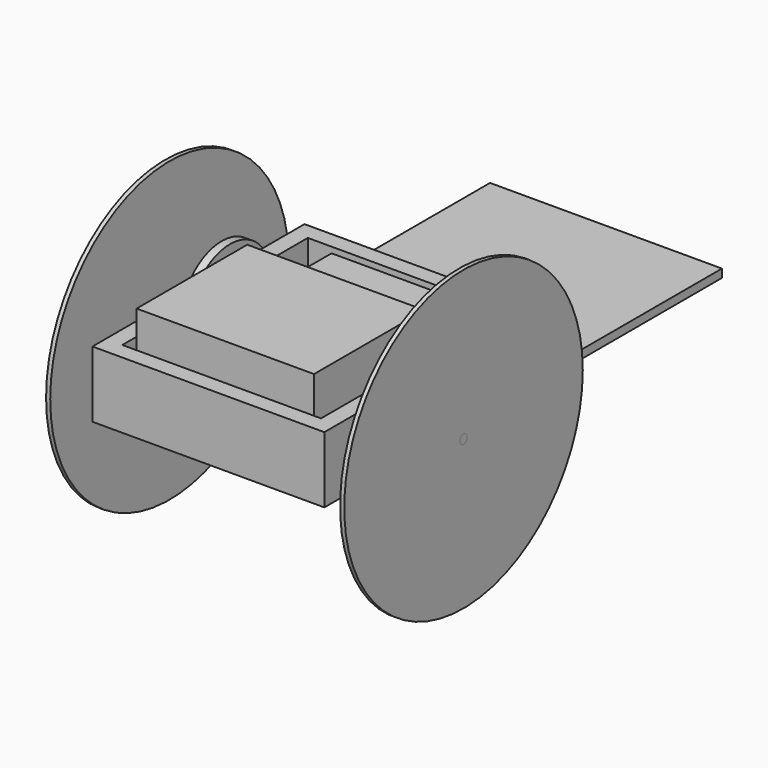
from build123d import *

# Parameters (mm, degrees)
F0_W           = 88.9
F0_H           = 101.6
F0_W_2         = 76.2
F0_H_2         = 88.9
F1_DEPTH       = 25.4
F2_DEPTH       = 3.175
F3_W           = 88.9
F3_H           = 3.175
F4_DEPTH       = 76.2
F5_W           = 47.999904
F5_H           = 25.0000008
F6_DEPTH       = 15.0114
F5_W_2         = 68.000118
F5_H_2         = 52.999894
F7_DEPTH       = 26.0096
F8_R           = 1.7859375
F9_DEPTH       = 6.35
F10_R          = 1.7859375
F11_DEPTH      = 6.35
F12_DEPTH      = 57.15
F12_DEPTH_BACK = 57.15
F15_R          = 57.15
F15_R_2        = 1.7859375
F16_DEPTH      = 1.5875
F17_R          = 57.15
F17_R_2        = 1.7859375
F18_DEPTH      = 1.5875
F20_R          = 1.7859375
F21_DEPTH      = 3.175
F22_R          = 5.0000027
F22_R_2        = 1.7859375
F23_DEPTH      = 3.175
F20_R_2        = 19.99996
F24_DEPTH      = 3.175
F25_DEPTH      = 3.175
F26_DEPTH      = 3.175


# Not quite as in the source:
# - a length typed as a fraction of an inch, garbled in the dataset ("3 / 203.2 mm" for 3/8 in), is restored


with BuildPart() as f1:
    # F0 (on Top) → F1 (new body)
    with BuildSketch(Plane.XY):
        Rectangle(F0_W, F0_H)
        Rectangle(F0_W_2, F0_H_2, mode=Mode.SUBTRACT)
    extrude(amount=F1_DEPTH)

    # F0 (on Top) → F2 (join)
    with BuildSketch(Plane.XY):
        Rectangle(F0_W_2, F0_H_2)
    extrude(amount=F2_DEPTH)

    # F8 (on face) → F9 (cut)
    with BuildSketch(Plane(origin=(-44.45, 0, 0), x_dir=(0, -1, 0), z_dir=(-1, 0, 0))):
        with Locations((0, 6.5484375)):
            Circle(F8_R)
    extrude(amount=-F9_DEPTH, mode=Mode.SUBTRACT)

    # F10 (on face) → F11 (cut)
    with BuildSketch(Plane.YZ.offset(44.45)):
        with Locations((0, 6.5484375)):
            Circle(F10_R)
    extrude(amount=-F11_DEPTH, mode=Mode.SUBTRACT)

    # F0 (on Top) → F26 (join)
    with BuildSketch(Plane.XY):
        with Locations((0, 95.25)):
            Rectangle(F0_W, F0_H_2)
    extrude(amount=F26_DEPTH)


with BuildPart() as f4:
    # F3 (on face) → F4 (new body)
    with BuildSketch(Plane.YZ.offset(-38.1)):
        with Locations((0, 10.715625)):
            Rectangle(F3_W, F3_H)
    extrude(amount=F4_DEPTH)


with BuildPart() as f6:
    # F5 (on face) → F6 (new body)
    with BuildSketch(Plane.XY.offset(12.303125)):
        with Locations((0, 25.7093309629)):
            Rectangle(F5_W, F5_H)
    extrude(amount=F6_DEPTH)


with BuildPart() as f7:
    # F5 (on face) → F7 (new body)
    with BuildSketch(Plane.XY.offset(12.303125)):
        with Locations((0, -16.2006690371)):
            Rectangle(F5_W_2, F5_H_2)
    extrude(amount=F7_DEPTH)


with BuildPart() as f12:
    # F8 (on face) → F12 (new body, two sides)
    with BuildSketch(Plane(origin=(-44.45, 0, 0), x_dir=(0, -1, 0), z_dir=(-1, 0, 0))) as f12_sk:
        with Locations((0, 6.5484375)):
            Circle(F8_R)
    extrude(amount=-F12_DEPTH)
    extrude(f12_sk.sketch, amount=F12_DEPTH_BACK)


with BuildPart() as f12_1:
    # F13: moved
    add(f12.part.moved(Location((38.1, 0, 0))))


with BuildPart() as f12_2:
    # F14: moved
    add(f12_1.part.moved(Location((6.35, 0, 0))))


with BuildPart() as f16:
    # F15 (on face) → F16 (new body)
    with BuildSketch(Plane.YZ.offset(57.15)):
        with Locations((0, 6.5484375)):
            Circle(F15_R)
        with Locations((0, 6.5484375)):
            Circle(F15_R_2, mode=Mode.SUBTRACT)
    extrude(amount=-F16_DEPTH)


with BuildPart() as f18:
    # F17 (on face) → F18 (new body)
    with BuildSketch(Plane(origin=(-57.15, 0, 0), x_dir=(0, -1, 0), z_dir=(-1, 0, 0))):
        with Locations((0, 6.5484375)):
            Circle(F17_R)
        with Locations((0, 6.5484375)):
            Circle(F17_R_2, mode=Mode.SUBTRACT)
    extrude(amount=-F18_DEPTH)


with BuildPart() as f21:
    # F20 (on face) → F21 (new body)
    with BuildSketch(Plane(origin=(55.5625, 0, 0), x_dir=(0, -1, 0), z_dir=(-1, 0, 0))):
        with BuildLine():
            ThreePointArc((-5.0000027, 6.5484375), (0, 1.5484348), (5.0000027, 6.5484375))
            ThreePointArc((5.0000027, 6.5484375), (0, 11.5484402), (-5.0000027, 6.5484375))
        make_face()
        with Locations((0, 6.5484375)):
            Circle(F20_R, mode=Mode.SUBTRACT)
    extrude(amount=F21_DEPTH)


with BuildPart() as f23:
    # F22 (on face) → F23 (new body)
    with BuildSketch(Plane.YZ.offset(-55.5625)):
        with Locations((0, 6.5484375)):
            Circle(F22_R)
        with Locations((0, 6.5484375)):
            Circle(F22_R_2, mode=Mode.SUBTRACT)
    extrude(amount=F23_DEPTH)


with BuildPart() as f24:
    # F20 (on face) → F24 (new body)
    with BuildSketch(Plane(origin=(55.5625, 0, 0), x_dir=(0, -1, 0), z_dir=(-1, 0, 0))):
        with Locations((-24.9999627, 6.5484375)):
            Circle(F20_R_2)
    extrude(amount=F24_DEPTH)


with BuildPart() as f25:
    # F22 (on face) → F25 (new body)
    with BuildSketch(Plane.YZ.offset(-55.5625)):
        with BuildLine():
            ThreePointArc((44.9999227, 6.5484375), (24.9999627, 26.5483975), (5.0000027, 6.5484375))
            ThreePointArc((5.0000027, 6.5484375), (24.9999627, -13.4515225), (44.9999227, 6.5484375))
        make_face()
    extrude(amount=F25_DEPTH)


solid = Compound([f1.part, f4.part, f6.part, f7.part, f12_2.part, f16.part, f18.part, f21.part, f23.part, f24.part, f25.part])
